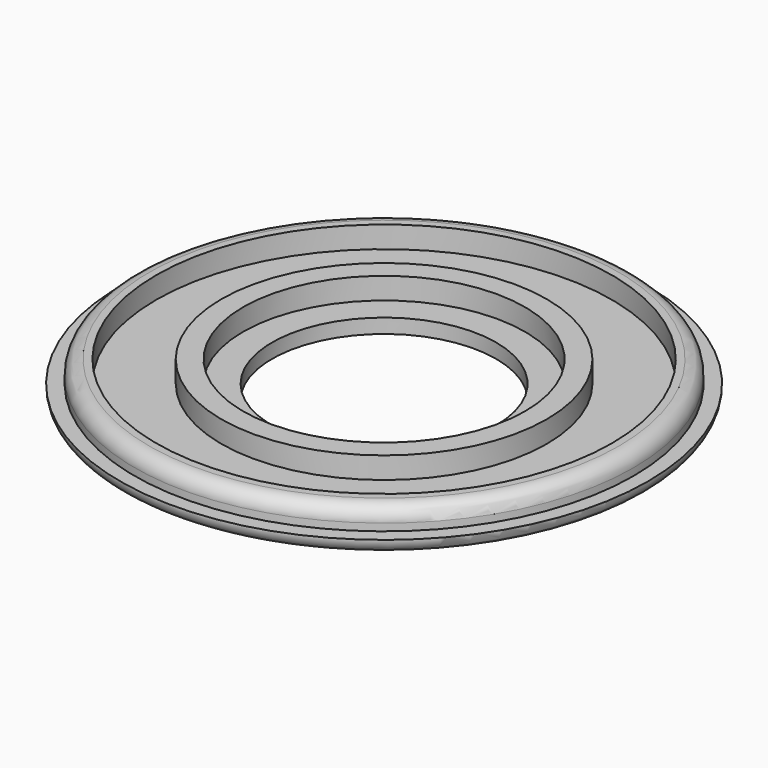
from build123d import *

# Parameters (mm, degrees)
F0_R     = 36.5
F0_R_2   = 34.5
F0_R_3   = 31.5
F0_R_4   = 22.5
F0_R_5   = 19.5
F1_DEPTH = 2
F2_DEPTH = 5
F3_R     = 1.99999
F4_R     = 2
F0_R_6   = 15.5
F5_DEPTH = 2


# Not quite as in the source:
# - a fillet or chamfer is up to 0.001 mm smaller than in the source, because OpenCascade refuses the exact size


with BuildPart() as f1:
    # F0 (on Top) → F1 (new body)
    with BuildSketch(Plane.XY):
        Circle(F0_R)
        Circle(F0_R_2, mode=Mode.SUBTRACT)
        Circle(F0_R_2)
        Circle(F0_R_3, mode=Mode.SUBTRACT)
        Circle(F0_R_3)
        Circle(F0_R_4, mode=Mode.SUBTRACT)
        Circle(F0_R_4)
        Circle(F0_R_5, mode=Mode.SUBTRACT)
    extrude(amount=F1_DEPTH)

    # F0 (on Top) → F2 (join)
    with BuildSketch(Plane.XY):
        Circle(F0_R_2)
        Circle(F0_R_3, mode=Mode.SUBTRACT)
        Circle(F0_R_4)
        Circle(F0_R_5, mode=Mode.SUBTRACT)
    extrude(amount=F2_DEPTH)

    # F3 (radius 2 in the source; OpenCascade refuses exactly that, so slightly less here)
    f3_edges = [f1.edges().sort_by_distance(p)[0] for p in [
        (-36.5, 0, 0),
    ]]
    fillet(f3_edges, radius=F3_R)

    # F4
    f4_edges = [f1.edges().sort_by_distance(p)[0] for p in [
        (-34.5, 0, 5),
    ]]
    fillet(f4_edges, radius=F4_R)

    # F0 (on Top) → F5 (join)
    with BuildSketch(Plane.XY):
        Circle(F0_R_5)
        Circle(F0_R_6, mode=Mode.SUBTRACT)
    extrude(amount=F5_DEPTH)


solid = f1.part
